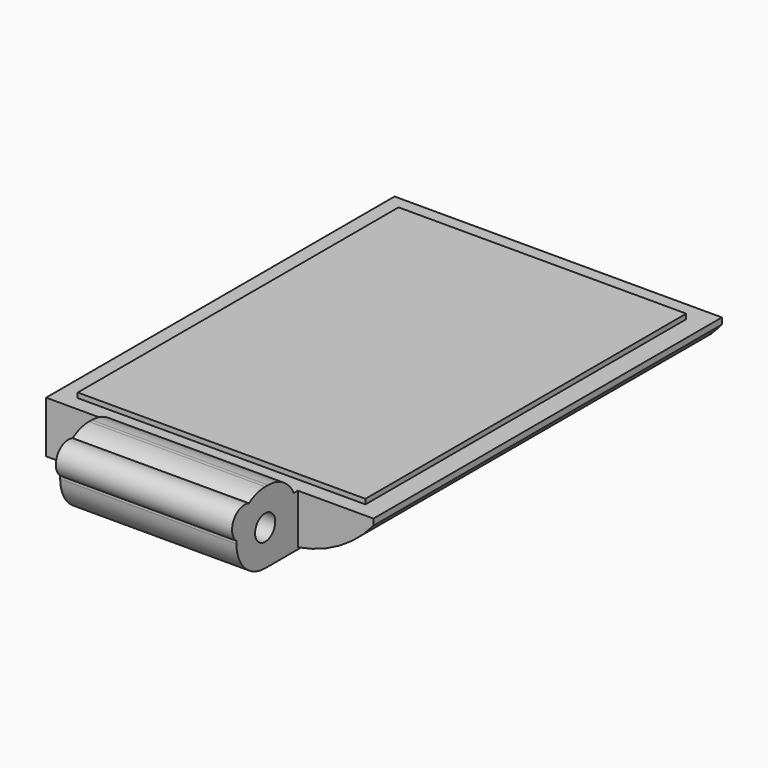
from build123d import *

# Parameters (mm, degrees)
F0_W         = 33.02
F0_H         = 44.45
F1_DEPTH     = 5.715
F2_W         = 17.78
F2_H         = 7.239
F3_DEPTH     = 7.239
F4_R         = 1.27
F5_DEPTH     = 19.05
F6_W         = 33.02
F6_H         = 44.45
F6_W_2       = 29.02
F6_H_2       = 40.45
F7_DEPTH     = 0.5
F9_DEPTH     = 33.02
F10_T1_DEPTH = 35.8775
F10_T3_DEPTH = 34.0243528649
F11_R        = 3.175
F12_DEPTH    = 1.27
F14_DEPTH    = 17.78
F15_W        = 7.62
F15_H        = 5.215
F16_DEPTH    = 0.508
F19_DEPTH    = 76.2


# Not quite as in the source:
# - a fillet or chamfer that OpenCascade refuses, or shapes differently, is made with other operations: its cross-section is extruded or revolved along the edge and cut away or added


with BuildPart() as f1:
    # F0 (on Top) → F1 (new body)
    with BuildSketch(Plane.XY):
        Rectangle(F0_W, F0_H)
    extrude(amount=F1_DEPTH)

    # F2 (on face) → F3 (join)
    with BuildSketch(Plane.XZ.offset(22.225)):
        with Locations((0, 3.6195)):
            Rectangle(F2_W, F2_H)
    extrude(amount=F3_DEPTH)

    # F4 (on face) → F5 (cut)
    with BuildSketch(Plane.YZ.offset(8.89)):
        with Locations((-25.8445, 3.6195)):
            Circle(F4_R)
    extrude(amount=-F5_DEPTH, mode=Mode.SUBTRACT)

    # F6 (on face) → F7 (cut)
    with BuildSketch(Plane.XY.offset(5.715)):
        Rectangle(F6_W, F6_H)
        Rectangle(F6_W_2, F6_H_2, mode=Mode.SUBTRACT)
    extrude(amount=-F7_DEPTH, mode=Mode.SUBTRACT)

    # F8 (on face) → F9 (join, through all)
    with BuildSketch(Plane.YZ.offset(16.51)):
        with BuildLine():
            Line((22.225, 3.175), (22.225, 0))
            ThreePointArc((22.225, 0), (23.8125, 1.5875), (22.225, 3.175))
        make_face()
    extrude(amount=-F9_DEPTH)

    # F10: fillet of radius 3.6195 on 3 edges, made by hand

    # F10_s2 → F10_t1 (cut)
    with BuildSketch(Plane.YZ.offset(-17.93875)):
        with BuildLine():
            ThreePointArc((-29.464, 3.6195), (-28.4038729945, 6.1788729945), (-25.8445, 7.239))
            Line((-25.8445, 7.239), (-25.8445, 7.31139))
            Line((-25.8445, 7.31139), (-29.53639, 7.31139))
            Line((-29.53639, 7.31139), (-29.53639, 3.6195))
            Line((-29.53639, 3.6195), (-29.464, 3.6195))
        make_face()
        with BuildLine():
            ThreePointArc((-25.8445, 0), (-28.4038729945, 1.0601270055), (-29.464, 3.6195))
            Line((-29.464, 3.6195), (-29.53639, 3.6195))
            Line((-29.53639, 3.6195), (-29.53639, -0.07239))
            Line((-29.53639, -0.07239), (-25.8445, -0.07239))
            Line((-25.8445, -0.07239), (-25.8445, 0))
        make_face()
    extrude(amount=F10_T1_DEPTH, mode=Mode.SUBTRACT)

    # F10_s4 → F10_t3 (cut)
    with BuildSketch(Plane.YZ.offset(-17.0121764325)):
        with BuildLine():
            ThreePointArc((-22.225, 5.215), (-23.5599912664, 6.6916077862), (-25.473870573, 7.239))
            Line((-25.473870573, 7.239), (-25.473870573, 7.31139))
            Line((-25.473870573, 7.31139), (-22.225, 7.31139))
            Line((-22.225, 7.31139), (-22.15261, 7.239))
            ThreePointArc((-22.15261, 7.239), (-22.15261, 6.227), (-22.1600225885, 5.24691))
            Line((-22.1600225885, 5.24691), (-22.225, 5.215))
        make_face()
    extrude(amount=F10_T3_DEPTH, mode=Mode.SUBTRACT)

    # F11 (on face) → F12 (cut)
    with BuildSketch(Plane(origin=(0, 0, 0), x_dir=(1, 0, 0), z_dir=(0, 0, -1))):
        with Locations((0, -17.78)):
            Circle(F11_R)
    extrude(amount=-F12_DEPTH, mode=Mode.SUBTRACT)

    # F13 (on face) → F14 (join)
    with BuildSketch(Plane.YZ.offset(8.89)):
        with BuildLine():
            ThreePointArc((-29.4532143561, 3.8987148746), (-28.979078949, 5.42925), (-27.8906643526, 6.6051308701))
            ThreePointArc((-27.8906643526, 6.6051308701), (-29.8039681461, 5.9055), (-29.4532143561, 3.8987148746))
        make_face()
    extrude(amount=-F14_DEPTH)

    # F15 (on face) → F16 (cut)
    with BuildSketch(Plane.XZ.offset(22.225)):
        with Locations((-12.7, 2.6075)):
            Rectangle(F15_W, F15_H)
        with Locations((12.7, 2.6075)):
            Rectangle(F15_W, F15_H)
    extrude(amount=-F16_DEPTH, mode=Mode.SUBTRACT)

    # F18 (on face) → F19 (cut)
    with BuildSketch(Plane.XZ.offset(21.717)):
        with BuildLine():
            ThreePointArc((16.51, 4.5832213708), (13.0932734681, 1.702037729), (8.89, 0.182915771))
            Line((8.89, 0.182915771), (8.89, 0))
            Line((8.89, 0), (16.51, 0))
            Line((16.51, 0), (16.51, 4.5832213708))
        make_face()
    extrude(amount=-F19_DEPTH, mode=Mode.SUBTRACT)


solid = f1.part
